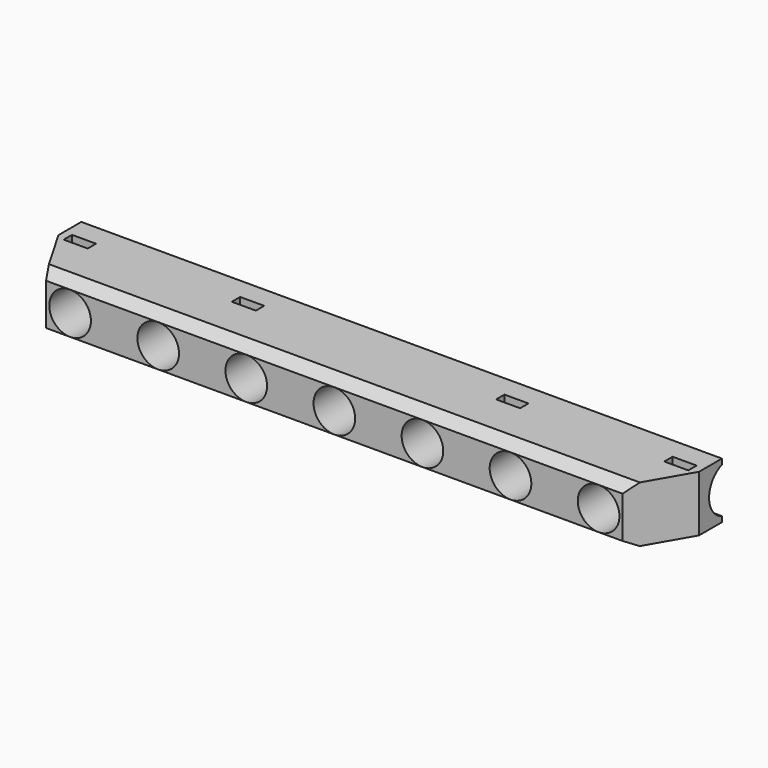
from build123d import *

# Parameters (mm, degrees)
F0_W          = 80
F0_H          = 7
F0_R          = 2.6
F1_DEPTH      = 11.5
F2_R          = 3
F3_DEPTH      = 5
F4_R          = 3
F5_DEPTH      = 80.001
F6_W          = 4
F6_H          = 3.5
F7_DEPTH      = 39
F7_DEPTH_BACK = 39
F8_SIZE2      = 6.9282032303
F8_SIZE       = 4
F9_SIZE2      = 1.558836
F9_SIZE       = 0.89999
F10_W         = 2
F10_H         = 10.311042398
F11_DEPTH     = 80.001
F12_R         = 3.5
F13_DEPTH     = 1.75
F14_T4_DEPTH  = 17.5408905874
F14_T9_DEPTH  = 17.5408905874
F15_W         = 3
F15_H         = 1.3
F16_DEPTH     = 7.0010001


# Not quite as in the source:
# - a fillet or chamfer that OpenCascade refuses, or shapes differently, is made with other operations: its cross-section is extruded or revolved along the edge and cut away or added
# - a fillet or chamfer is up to 0.001 mm smaller than in the source, because OpenCascade refuses the exact size


with BuildPart() as f1:
    # F0 (on Front) → F1 (new body)
    with BuildSketch(Plane.XZ):
        Rectangle(F0_W, F0_H)
        with Locations((-33, 0)):
            Circle(F0_R, mode=Mode.SUBTRACT)
        with Locations((-22, 0)):
            Circle(F0_R, mode=Mode.SUBTRACT)
        with Locations((-11, 0)):
            Circle(F0_R, mode=Mode.SUBTRACT)
        Circle(F0_R, mode=Mode.SUBTRACT)
        with Locations((11, 0)):
            Circle(F0_R, mode=Mode.SUBTRACT)
        with Locations((22, 0)):
            Circle(F0_R, mode=Mode.SUBTRACT)
        with Locations((33, 0)):
            Circle(F0_R, mode=Mode.SUBTRACT)
    extrude(amount=F1_DEPTH)

    # F2 (on face) → F3 (cut)
    with BuildSketch(Plane(origin=(0, 0, 0), x_dir=(-1, 0, 0), z_dir=(0, 1, 0))):
        Circle(F2_R)
        with Locations((11, 0)):
            Circle(F2_R)
        with Locations((22, 0)):
            Circle(F2_R)
        with Locations((33, 0)):
            Circle(F2_R)
        with Locations((-11, 0)):
            Circle(F2_R)
        with Locations((-22, 0)):
            Circle(F2_R)
        with Locations((-33, 0)):
            Circle(F2_R)
    extrude(amount=-F3_DEPTH, mode=Mode.SUBTRACT)

    # F4 (on face) → F5 (cut, through all)
    with BuildSketch(Plane(origin=(-40, 0, 0), x_dir=(0, -1, 0), z_dir=(-1, 0, 0))):
        Circle(F4_R)
    extrude(amount=-F5_DEPTH, mode=Mode.SUBTRACT)

    # F6 (on Right) → F7 (cut, two sides)
    with BuildSketch(Plane.YZ) as f7_sk:
        with Locations((-3, 0)):
            Rectangle(F6_W, F6_H)
    extrude(amount=-F7_DEPTH, mode=Mode.SUBTRACT)
    extrude(f7_sk.sketch, amount=F7_DEPTH_BACK, mode=Mode.SUBTRACT)

    # F8
    f8_edges = [f1.edges().sort_by_distance(p)[0] for p in [
        (-40, -11.5, 0),
        (40, -11.5, 0),
    ]]
    f8_side = f1.faces().sort_by_distance((39.196943, -11.5, 0))[0]
    chamfer(f8_edges, length=F8_SIZE, length2=F8_SIZE2, reference=f8_side)

    # F9 (size 0.9 and 1.5588457268 in the source; OpenCascade refuses exactly that, so slightly less here)
    f9_edges = [f1.edges().sort_by_distance(p)[0] for p in [
        (0, -11.5, 3.5),
        (0, -11.5, -3.5),
    ]]
    f9_side = f1.faces().sort_by_distance((0, -11.5, 2.776605))[0]
    chamfer(f9_edges, length=F9_SIZE, length2=F9_SIZE2, reference=f9_side)

    # F10 (on face) → F11 (cut, through all)
    with BuildSketch(Plane(origin=(-40, 0, 0), x_dir=(0, -1, 0), z_dir=(-1, 0, 0))):
        Rectangle(F10_W, F10_H)
    extrude(amount=-F11_DEPTH, mode=Mode.SUBTRACT)

    # F12 (on face) → F13 (cut, through all)
    with BuildSketch(Plane(origin=(0, 0, -3.5), x_dir=(1, 0, 0), z_dir=(0, 0, -1))):
        with Locations((0, 1)):
            Circle(F12_R)
    extrude(amount=-F13_DEPTH, mode=Mode.SUBTRACT)

    # F14: fillet of radius 5 on 2 edges, made by hand


with BuildPart() as f14_tool2:
    # F14_s3 → F14_t4 (new body)
    with BuildSketch(Plane.XY.offset(5.6062317314)):
        with BuildLine():
            ThreePointArc((-6.8738635424, -1), (-4.60515051, -1.5443360566), (-2.8304143998, -3.0588235294))
            ThreePointArc((-2.8304143998, -3.0588235294), (-3.3283967912, -2.0824854735), (-3.5, -1))
            Line((-3.5, -1), (-6.8738635424, -1))
        make_face()
    extrude(amount=-F14_T4_DEPTH)

    split(bisect_by=Plane.XY.offset(1.75), keep=Keep.BOTTOM)


with BuildPart() as f1_1:
    add(f1.part)

    # F14_t1: cut F14_tool2
    add(f14_tool2.part, mode=Mode.SUBTRACT)


with BuildPart() as f14_tool7:
    # F14_s8 → F14_t9 (new body)
    with BuildSketch(Plane.XY.offset(-11.9346588561)):
        with BuildLine():
            ThreePointArc((2.8304143998, -3.0588235294), (4.60515051, -1.5443360566), (6.8738635424, -1))
            Line((6.8738635424, -1), (3.5, -1))
            ThreePointArc((3.5, -1), (3.3283967912, -2.0824854735), (2.8304143998, -3.0588235294))
        make_face()
    extrude(amount=F14_T9_DEPTH)

    split(bisect_by=Plane.XY.offset(1.75), keep=Keep.BOTTOM)


with BuildPart() as f1_2:
    add(f1_1.part)

    # F14_t6: cut F14_tool7
    add(f14_tool7.part, mode=Mode.SUBTRACT)

    # F15 (on face) → F16 (cut, through all)
    with BuildSketch(Plane.XY.offset(3.5)):
        with Locations((37.5, -4.35)):
            Rectangle(F15_W, F15_H)
        with Locations((16.5, -4.35)):
            Rectangle(F15_W, F15_H)
        with Locations((-16.5, -4.35)):
            Rectangle(F15_W, F15_H)
        with Locations((-37.5, -4.35)):
            Rectangle(F15_W, F15_H)
    extrude(amount=-F16_DEPTH, mode=Mode.SUBTRACT)


solid = f1_2.part
